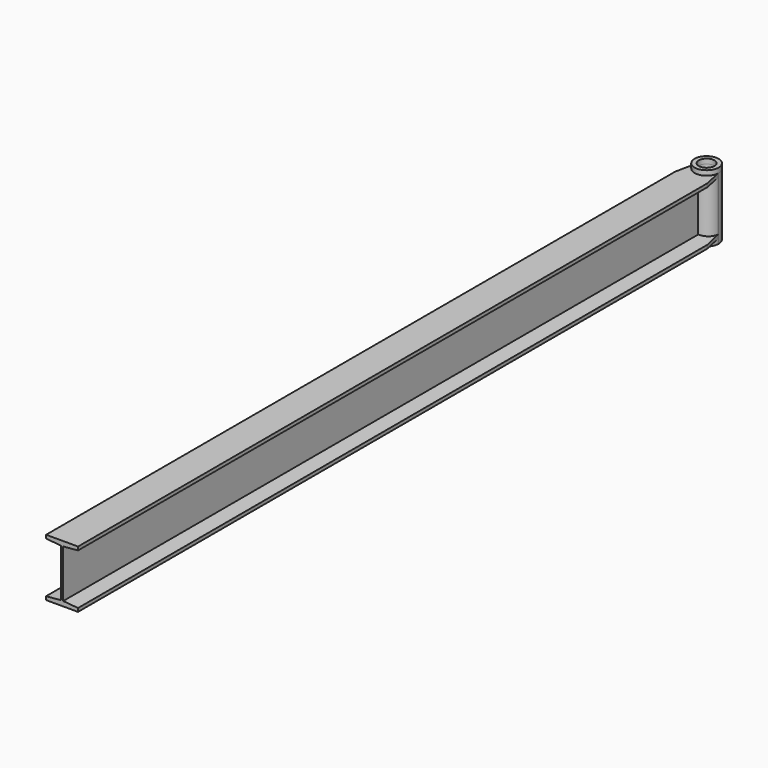
from build123d import *

# Parameters (mm, degrees)
F1_DEPTH      = 1066.8
F2_T4_DEPTH   = 2133.6
F2_T9_DEPTH   = 2133.6
F3_T4_DEPTH   = 2133.6
F3_T9_DEPTH   = 2133.6
F5_DEPTH      = 165.1
F5_DEPTH_BACK = 12.7
F6_R          = 20.6375
F7_DEPTH      = 165.101
F9_DEPTH      = 165.101


# Not quite as in the source:
# - a fillet or chamfer that OpenCascade refuses, or shapes differently, is made with other operations: its cross-section is extruded or revolved along the edge and cut away or added


with BuildPart() as f1:
    # F0 (on Front) → F1 (new body, symmetric)
    with BuildSketch(Plane.XZ):
        Polygon((39.37, 143.2814), (0, 143.2814), (0, 134.1628), (39.37, 134.1628), (39.37, 0), (0, 0), (0, -9.1186), (84.6328, -9.1186), (84.6328, 0), (45.2628, 0), (45.2628, 134.1628), (84.6328, 134.1628), (84.6328, 143.2814), (45.2628, 143.2814), align=None)
    extrude(amount=F1_DEPTH, both=True)

    # F2: chamfer of 3.44678 x 39.3968756761 on 2 edges, made by hand


with BuildPart() as f2_tool2:
    # F2_s3 → F2_t4 (new body)
    with BuildSketch(Plane.XZ.offset(-1066.8)):
        Polygon((39.37, 130.71602), (-0.0268756761, 134.1628), (39.37, 134.1628), align=None)
    extrude(amount=F2_T4_DEPTH)

    split(bisect_by=Plane.YZ, keep=Keep.TOP)


with BuildPart() as f1_1:
    add(f1.part)

    # F2_t1: union F2_tool2
    add(f2_tool2.part)


with BuildPart() as f2_tool7:
    # F2_s8 → F2_t9 (new body)
    with BuildSketch(Plane.XZ.offset(-1066.8)):
        Polygon((45.2628, 3.44678), (84.6596756761, 0), (45.2628, 0), align=None)
    extrude(amount=F2_T9_DEPTH)

    split(bisect_by=Plane.YZ.offset(84.6328), keep=Keep.BOTTOM)


with BuildPart() as f1_2:
    add(f1_1.part)

    # F2_t6: union F2_tool7
    add(f2_tool7.part)

    # F3: chamfer of 3.45186 x 39.4549403418 on 2 edges, made by hand


with BuildPart() as f3_tool2:
    # F3_s3 → F3_t4 (new body)
    with BuildSketch(Plane.XZ.offset(-1066.8)):
        Polygon((-0.0849403418, 0), (39.37, 3.45186), (39.37, 0), align=None)
    extrude(amount=F3_T4_DEPTH)

    split(bisect_by=Plane.YZ, keep=Keep.TOP)


with BuildPart() as f1_3:
    add(f1_2.part)

    # F3_t1: union F3_tool2
    add(f3_tool2.part)


with BuildPart() as f3_tool7:
    # F3_s8 → F3_t9 (new body)
    with BuildSketch(Plane.XZ.offset(-1066.8)):
        Polygon((84.7177403418, 134.1628), (45.2628, 130.71094), (45.2628, 134.1628), align=None)
    extrude(amount=F3_T9_DEPTH)

    split(bisect_by=Plane.YZ.offset(84.6328), keep=Keep.BOTTOM)


with BuildPart() as f1_4:
    add(f1_3.part)

    # F3_t6: union F3_tool7
    add(f3_tool7.part)

    # F6 (on face) → F7 (cut, through all)
    with BuildSketch(Plane.XY.offset(143.2814)):
        with Locations((42.3164, 1066.8)):
            Circle(F6_R)
    extrude(amount=-F7_DEPTH, mode=Mode.SUBTRACT)


with BuildPart() as f5:
    # F4 (on face) → F5 (new body, two sides)
    with BuildSketch(Plane.XY.offset(143.2814)) as f5_sk:
        with BuildLine():
            ThreePointArc((10.5664, 1066.8), (42.3164, 1035.05), (74.0664, 1066.8))
            Line((74.0664, 1066.8), (62.9539, 1066.8))
            ThreePointArc((62.9539, 1066.8), (42.3164, 1046.1625), (21.6789, 1066.8))
            Line((21.6789, 1066.8), (10.5664, 1066.8))
        make_face()
        with BuildLine():
            Line((62.9539, 1066.8), (74.0664, 1066.8))
            ThreePointArc((74.0664, 1066.8), (42.3164, 1098.55), (10.5664, 1066.8))
            Line((10.5664, 1066.8), (21.6789, 1066.8))
            ThreePointArc((21.6789, 1066.8), (42.3164, 1087.4375), (62.9539, 1066.8))
        make_face()
    extrude(amount=-F5_DEPTH)
    extrude(f5_sk.sketch, amount=F5_DEPTH_BACK)


with BuildPart() as f9_tool:
    # F8 (on face) → F9 (new body, through all)
    with BuildSketch(Plane.XY.offset(143.2814)):
        Polygon((0, 1016), (10.83945, 1066.8), (0, 1066.8), align=None)
        Polygon((84.6328, 1016), (84.6328, 1066.8), (73.79335, 1066.8), align=None)
    extrude(amount=-F9_DEPTH)


with BuildPart() as f1_5:
    add(f1_4.part)

    # F9: cut by f9_tool
    add(f9_tool.part, mode=Mode.SUBTRACT)


with BuildPart() as f5_1:
    add(f5.part)

    # F9: cut by f9_tool
    add(f9_tool.part, mode=Mode.SUBTRACT)


solid = Compound([f1_5.part, f5_1.part])
